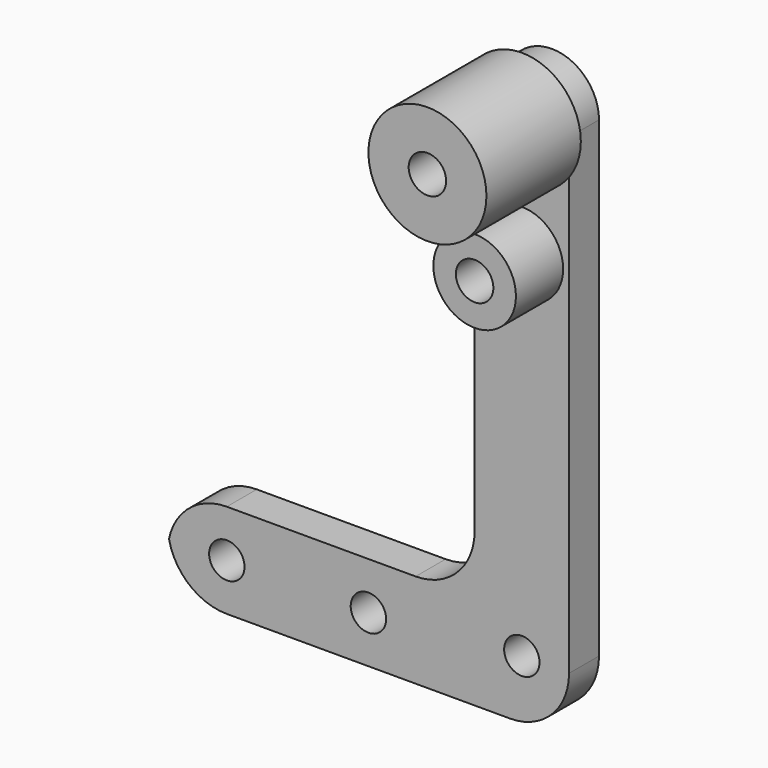
from build123d import *

# Parameters (mm, degrees)
F0_R        = 1.5
F0_W        = 8
F0_H        = 8
F0_W_2      = 26
F1_DEPTH    = 3.175
F2_T1_DEPTH = 3.175
F2_T3_DEPTH = 28.175
F3_R        = 5
F3_R_2      = 1.5875
F4_DEPTH    = 10
F5_R        = 3.5
F5_R_2      = 1.5875
F6_DEPTH    = 5


# Not quite as in the source:
# - a fillet or chamfer that OpenCascade refuses, or shapes differently, is made with other operations: its cross-section is extruded or revolved along the edge and cut away or added
# - a length typed as a fraction of an inch, garbled in the dataset ("3 / 203.2 mm" for 3/8 in), is restored


with BuildPart() as f1:
    # F0 (on Front) → F1 (new body)
    with BuildSketch(Plane.XZ):
        with BuildLine():
            ThreePointArc((4, 10), (0, 14), (-4, 10))
            ThreePointArc((-4, 10), (0, 6), (4, 10))
        make_face()
        with Locations((0, 10)):
            Circle(F0_R, mode=Mode.SUBTRACT)
        with BuildLine():
            ThreePointArc((4, 10), (0, 6), (-4, 10))
            Line((-4, 10), (-4, -27))
            Line((-4, -27), (4, -27))
            Line((4, -27), (4, 10))
        make_face()
        Circle(F0_R, mode=Mode.SUBTRACT)
        with Locations((0, -31)):
            Rectangle(F0_W, F0_H)
        with Locations((0, -30)):
            Circle(F0_R, mode=Mode.SUBTRACT)
        with Locations((-17, -31)):
            Rectangle(F0_W_2, F0_H)
        with Locations((-25, -31)):
            Circle(F0_R, mode=Mode.SUBTRACT)
        with Locations((-13, -31)):
            Circle(F0_R, mode=Mode.SUBTRACT)
    extrude(amount=F1_DEPTH)

    # F2: fillet of radius 5 on 4 edges, made by hand

    # F2_s2 → F2_t1 (join)
    with BuildSketch(Plane.XZ):
        with BuildLine():
            ThreePointArc((-4, -22), (-5.4644660941, -25.5355339059), (-9, -27))
            Line((-9, -27), (-4, -27))
            Line((-4, -27), (-4, -22))
        make_face()
    extrude(amount=F2_T1_DEPTH)

    # F2_s4 → F2_t3 (cut)
    with BuildSketch(Plane.XZ.offset(-12.5)):
        with BuildLine():
            ThreePointArc((4, -30), (2.5355339059, -33.5355339059), (-1, -35))
            Line((-1, -35), (4, -35))
            Line((4, -35), (4, -30))
        make_face()
        with BuildLine():
            ThreePointArc((-25, -27), (-28.5355339059, -28.4644660941), (-30, -32))
            Line((-30, -32), (-30, -27))
            Line((-30, -27), (-25, -27))
        make_face()
        with BuildLine():
            ThreePointArc((-25, -35), (-28.5355339059, -33.5355339059), (-30, -30))
            Line((-30, -30), (-30, -35))
            Line((-30, -35), (-25, -35))
        make_face()
    extrude(amount=F2_T3_DEPTH, mode=Mode.SUBTRACT)


with BuildPart() as f4:
    # F3 (on face) → F4 (new body)
    with BuildSketch(Plane.XZ.offset(3.175)):
        with Locations((0, 10)):
            Circle(F3_R)
        with Locations((0, 10)):
            Circle(F3_R_2, mode=Mode.SUBTRACT)
    extrude(amount=F4_DEPTH)


with BuildPart() as f6:
    # F5 (on face) → F6 (new body)
    with BuildSketch(Plane.XZ.offset(3.175)):
        Circle(F5_R)
        Circle(F5_R_2, mode=Mode.SUBTRACT)
    extrude(amount=F6_DEPTH)


solid = Compound([f1.part, f4.part, f6.part])
